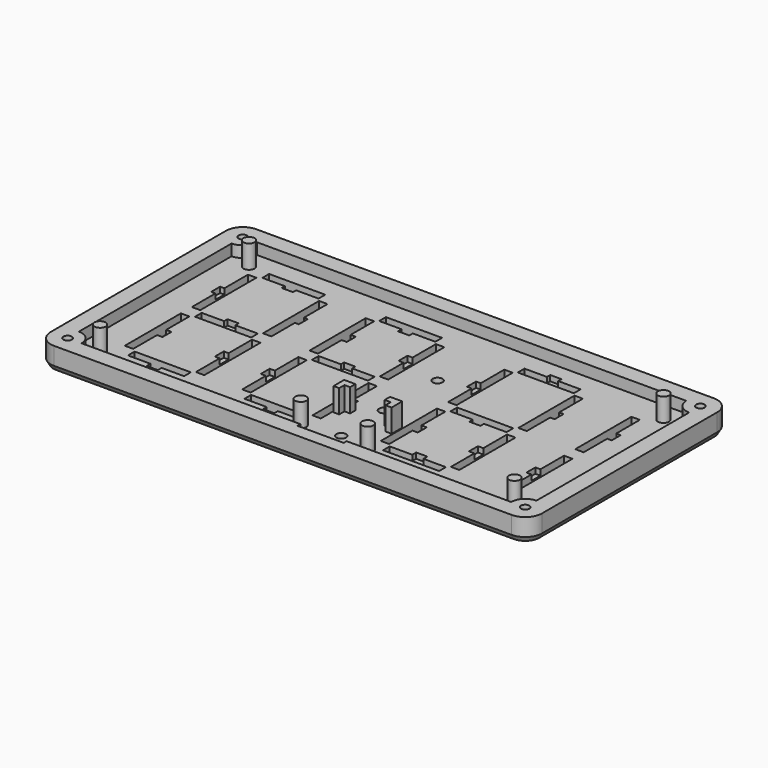
from build123d import *

# Parameters (mm, degrees)
F0_W     = 175
F0_H     = 90
F0_R     = 1.5
F0_R_2   = 2
F0_R_3   = 1.75
F0_W_2   = 16.51
F0_H_2   = 1.3014607364
F0_W_3   = 1.9210205078
F0_H_3   = 4
F0_W_4   = 1.9112368478
F0_W_5   = 1.867620334
F0_W_6   = 1.8335093537
F0_W_7   = 1.8196914813
F0_W_8   = 1.798794187
F0_H_4   = 3.9840501759
F0_W_9   = 1.7908662094
F0_W_10  = 4
F0_H_5   = 1.748018801
F0_W_11  = 1.7107389867
F0_H_6   = 1.7050467432
F0_W_12  = 1.6551189721
F0_H_7   = 1.612730462
F0_W_13  = 1.6000587711
F0_H_8   = 4.0289216264
F0_W_14  = 1.5901946127
F0_H_9   = 1.5753317512
F0_H_10  = 1.5676104019
F0_W_15  = 1.5668362754
F0_W_16  = 1.5211995589
F0_H_11  = 1.4929155913
F0_H_12  = 1.4762649832
F0_H_13  = 1.4190260208
F0_H_14  = 1.4116684069
F0_W_17  = 1.3783299625
F1_DEPTH = 4
F2_DEPTH = 4
F3_DEPTH = 4
F4_DEPTH = 2
F5_R     = 6
F6_SIZE2 = 1.7320508076
F6_SIZE  = 1
F8_DEPTH = 8.25


# Not quite as in the source:
# - a feature names something its author has since deleted; it is built from what else it names


with BuildPart() as f1:
    # F0 (on Top) → F1 (new body)
    with BuildSketch(Plane.XY):
        Rectangle(F0_W, F0_H)
        with Locations((-81.5, -39)):
            Circle(F0_R, mode=Mode.SUBTRACT)
        with Locations((81.5, -39)):
            Circle(F0_R, mode=Mode.SUBTRACT)
        with BuildLine():
            Line((-81.5, -34), (-81.5, 34))
            ThreePointArc((-81.5, 34), (-77.9644660941, 35.4644660941), (-76.5, 39))
            Line((-76.5, 39), (76.5, 39))
            ThreePointArc((76.5, 39), (77.9644660941, 35.4644660941), (81.5, 34))
            Line((81.5, 34), (81.5, -34))
            ThreePointArc((81.5, -34), (77.9644660941, -35.4644660941), (76.5, -39))
            Line((76.5, -39), (17.9069533545, -39))
            Line((17.9069533545, -39), (17.9069533545, -40.3014607364))
            Line((17.9069533545, -40.3014607364), (1.3969533545, -40.3014607364))
            Line((1.3969533545, -40.3014607364), (1.3969533545, -39))
            Line((1.3969533545, -39), (-76.5, -39))
            ThreePointArc((-76.5, -39), (-77.9644660941, -35.4644660941), (-81.5, -34))
        make_face(mode=Mode.SUBTRACT)
        with Locations((-81.5, 39)):
            Circle(F0_R, mode=Mode.SUBTRACT)
        with Locations((81.5, 39)):
            Circle(F0_R, mode=Mode.SUBTRACT)
        with BuildLine():
            ThreePointArc((-76.5, 39), (-77.9644660941, 35.4644660941), (-81.5, 34))
            Line((-81.5, 34), (-81.5, -34))
            ThreePointArc((-81.5, -34), (-77.9644660941, -35.4644660941), (-76.5, -39))
            Line((-76.5, -39), (1.3969533545, -39))
            Line((1.3969533545, -39), (17.9069533545, -39))
            Line((17.9069533545, -39), (76.5, -39))
            ThreePointArc((76.5, -39), (77.9644660941, -35.4644660941), (81.5, -34))
            Line((81.5, -34), (81.5, 34))
            ThreePointArc((81.5, 34), (77.9644660941, 35.4644660941), (76.5, 39))
            Line((76.5, 39), (-76.5, 39))
        make_face()
        with Locations((-74.491012668, -33.333260566)):
            Circle(F0_R_2, mode=Mode.SUBTRACT)
        Polygon((-66.6752069294, -27.6686349213), (-46.6752069294, -27.6686349213), (-46.6752069294, -30.6686349213), (-54.6752069294, -30.6686349213), (-54.6752069294, -32.3736816645), (-58.6752069294, -32.3736816645), (-58.6752069294, -30.6686349213), (-66.6752069294, -30.6686349213), align=None, mode=Mode.SUBTRACT)
        Polygon((-25.0613520422, -27.8102330678), (-5.0613520422, -27.8102330678), (-5.0613520422, -30.8102330678), (-13.1632021666, -30.8102330678), (-13.1632021666, -32.4229635298), (-17.1632021666, -32.4229635298), (-17.1632021666, -30.8102330678), (-25.0613520422, -30.8102330678), align=None, mode=Mode.SUBTRACT)
        with Locations((-2.9774932191, -33.333260566)):
            Circle(F0_R_2, mode=Mode.SUBTRACT)
        Polygon((-68.0133168949, -16.0233359784), (-68.0133168949, -26.6686349213), (-71.0133168949, -26.6686349213), (-71.0133168949, -1.6686349213), (-68.0133168949, -1.6686349213), (-68.0133168949, -12.0233359784), (-66.1020800471, -12.0233359784), (-66.1020800471, -16.0233359784), align=None, mode=Mode.SUBTRACT)
        Polygon((-45.6752069294, -12.0996839404), (-45.6752069294, -1.6686349213), (-42.6752069294, -1.6686349213), (-42.6752069294, -26.6686349213), (-45.6752069294, -26.6686349213), (-45.6752069294, -16.0996839404), (-47.3859459162, -16.0996839404), (-47.3859459162, -12.0996839404), align=None, mode=Mode.SUBTRACT)
        Polygon((-29.0613520422, -1.8102330678), (-26.0613520422, -1.8102330678), (-26.0613520422, -26.8102330678), (-29.0613520422, -26.8102330678), (-29.0613520422, -16.2864062117), (-30.8810435236, -16.2864062117), (-30.8810435236, -12.2864062117), (-29.0613520422, -12.2864062117), align=None, mode=Mode.SUBTRACT)
        Polygon((-4.0613520422, -26.8102330678), (-4.0613520422, -1.8102330678), (-1.0613520422, -1.8102330678), (-1.0613520422, -12.2331848519), (0.5054842331, -12.2331848519), (0.5054842331, -16.2331848519), (-1.0613520422, -16.2331848519), (-1.0613520422, -26.8102330678), align=None, mode=Mode.SUBTRACT)
        with Locations((9.8969533545, -31.4114607364)):
            Circle(F0_R_3, mode=Mode.SUBTRACT)
        with Locations((20.8698699123, -33.333260566)):
            Circle(F0_R_2, mode=Mode.SUBTRACT)
        Polygon((36.4340835214, -27.958609998), (44.4077534974, -27.958609998), (44.4077534974, -30.958609998), (24.4077534974, -30.958609998), (24.4077534974, -27.958609998), (32.4340835214, -27.958609998), (32.4340835214, -26.210591197), (36.4340835214, -26.210591197), align=None, mode=Mode.SUBTRACT)
        with Locations((73.1534102804, -33.333260566)):
            Circle(F0_R_2, mode=Mode.SUBTRACT)
        Polygon((1.3969533545, -19.3464607364), (1.3969533545, -21.7163469642), (-0.608429326, -21.7163469642), (-0.608429326, -16.9765745085), (3.4023360349, -16.9765745085), (3.4023360349, -19.3464607364), align=None, mode=Mode.SUBTRACT)
        Polygon((17.9069533545, -21.7163469642), (17.9069533545, -19.3464607364), (15.7326646149, -19.3464607364), (15.7326646149, -16.9765745085), (20.081242094, -16.9765745085), (20.081242094, -21.7163469642), align=None, mode=Mode.SUBTRACT)
        with Locations((9.6294777468, -12.0452046394)):
            Circle(F0_R_3, mode=Mode.SUBTRACT)
        Polygon((20.4077534974, -26.958609998), (20.4077534974, -1.958609998), (23.4077534974, -1.958609998), (23.4077534974, -12.5651864777), (25.2753738314, -12.5651864777), (25.2753738314, -16.5651864777), (23.4077534974, -16.5651864777), (23.4077534974, -26.958609998), align=None, mode=Mode.SUBTRACT)
        Polygon((24.4077534974, 2.041390002), (44.4077534974, 2.041390002), (44.4077534974, -0.958609998), (36.3806852102, -0.958609998), (36.3806852102, -2.5262203999), (32.3806852102, -2.5262203999), (32.3806852102, -0.958609998), (24.4077534974, -0.958609998), align=None, mode=Mode.SUBTRACT)
        Polygon((45.4077534974, -12.5448077023), (45.4077534974, -1.958609998), (48.4077534974, -1.958609998), (48.4077534974, -26.958609998), (45.4077534974, -26.958609998), (45.4077534974, -16.5448077023), (43.4867329895, -16.5448077023), (43.4867329895, -12.5448077023), align=None, mode=Mode.SUBTRACT)
        Polygon((65.7603075275, -12.5448077023), (65.7603075275, -2.0368327902), (68.7603075275, -2.0368327902), (68.7603075275, -27.0368327902), (65.7603075275, -27.0368327902), (65.7603075275, -16.5288578782), (63.9615133405, -16.5288578782), (63.9615133405, -12.5448077023), align=None, mode=Mode.SUBTRACT)
        Polygon((-54.6752069294, 2.1897669322), (-46.6752069294, 2.1897669322), (-46.6752069294, -0.8102330678), (-66.6752069294, -0.8102330678), (-66.6752069294, 2.1897669322), (-58.6752069294, 2.1897669322), (-58.6752069294, 3.6826825235), (-54.6752069294, 3.6826825235), align=None, mode=Mode.SUBTRACT)
        Polygon((-68.0133168949, 28.1897669322), (-68.0133168949, 3.1897669322), (-71.0133168949, 3.1897669322), (-71.0133168949, 13.6897669322), (-72.5345164537, 13.6897669322), (-72.5345164537, 17.6897669322), (-71.0133168949, 17.6897669322), (-71.0133168949, 28.1897669322), align=None, mode=Mode.SUBTRACT)
        Polygon((-13.103722319, 2.1897669322), (-5.0613520422, 2.1897669322), (-5.0613520422, -0.8102330678), (-25.0613520422, -0.8102330678), (-25.0613520422, 2.1897669322), (-17.103722319, 2.1897669322), (-17.103722319, 3.6014353391), (-13.103722319, 3.6014353391), align=None, mode=Mode.SUBTRACT)
        Polygon((-42.6752069294, 13.6755983604), (-42.6752069294, 3.1897669322), (-45.6752069294, 3.1897669322), (-45.6752069294, 28.1897669322), (-42.6752069294, 28.1897669322), (-42.6752069294, 17.6755983604), (-41.296876967, 17.6755983604), (-41.296876967, 13.6755983604), align=None, mode=Mode.SUBTRACT)
        Polygon((-29.0613520422, 28.1897669322), (-26.0613520422, 28.1897669322), (-26.0613520422, 17.6864017023), (-24.2278426886, 17.6864017023), (-24.2278426886, 13.6864017023), (-26.0613520422, 13.6864017023), (-26.0613520422, 3.1897669322), (-29.0613520422, 3.1897669322), align=None, mode=Mode.SUBTRACT)
        Polygon((-4.0613520422, 17.7803005055), (-4.0613520422, 28.1897669322), (-1.0613520422, 28.1897669322), (-1.0613520422, 3.1897669322), (-4.0613520422, 3.1897669322), (-4.0613520422, 13.7803005055), (-5.8522182517, 13.7803005055), (-5.8522182517, 17.7803005055), align=None, mode=Mode.SUBTRACT)
        with Locations((-73.842048645, 32.1897669322)):
            Circle(F0_R_2, mode=Mode.SUBTRACT)
        Polygon((-46.6752069294, 32.1897669322), (-46.6752069294, 29.1897669322), (-54.6752069294, 29.1897669322), (-54.6752069294, 27.7707409114), (-58.6752069294, 27.7707409114), (-58.6752069294, 29.1897669322), (-66.6752069294, 29.1897669322), (-66.6752069294, 32.1897669322), align=None, mode=Mode.SUBTRACT)
        Polygon((-5.0613520422, 32.1897669322), (-5.0613520422, 29.1897669322), (-13.1001572162, 29.1897669322), (-13.1001572162, 27.614435181), (-17.1001572162, 27.614435181), (-17.1001572162, 29.1897669322), (-25.0613520422, 29.1897669322), (-25.0613520422, 32.1897669322), align=None, mode=Mode.SUBTRACT)
        with Locations((10.0254695863, 11.318275705)):
            Circle(F0_R_3, mode=Mode.SUBTRACT)
        Polygon((23.4077534974, 28.041390002), (23.4077534974, 3.041390002), (20.4077534974, 3.041390002), (20.4077534974, 13.5473189875), (18.7526345253, 13.5473189875), (18.7526345253, 17.5473189875), (20.4077534974, 17.5473189875), (20.4077534974, 28.041390002), align=None, mode=Mode.SUBTRACT)
        Polygon((48.4077534974, 3.041390002), (45.4077534974, 3.041390002), (45.4077534974, 28.041390002), (48.4077534974, 28.041390002), (48.4077534974, 17.4776280229), (49.9979481101, 17.4776280229), (49.9979481101, 13.4776280229), (48.4077534974, 13.4776280229), align=None, mode=Mode.SUBTRACT)
        Polygon((68.7603075275, 2.9631672098), (65.7603075275, 2.9631672098), (65.7603075275, 27.9631672098), (68.7603075275, 27.9631672098), (68.7603075275, 17.4776280229), (70.3603662986, 17.4776280229), (70.3603662986, 13.4487063966), (68.7603075275, 13.4487063966), align=None, mode=Mode.SUBTRACT)
        Polygon((36.4043445289, 32.041390002), (44.4077534974, 32.041390002), (44.4077534974, 29.041390002), (24.4077534974, 29.041390002), (24.4077534974, 32.041390002), (32.4043445289, 32.041390002), (32.4043445289, 33.5176549852), (36.4043445289, 33.5176549852), align=None, mode=Mode.SUBTRACT)
        with Locations((73.8023817539, 32.1897669322)):
            Circle(F0_R_2, mode=Mode.SUBTRACT)
        Polygon((-1.0613520422, 28.1897669322), (-4.0613520422, 28.1897669322), (-4.0613520422, 17.7803005055), (-4.0613520422, 13.7803005055), (-4.0613520422, 3.1897669322), (-1.0613520422, 3.1897669322), align=None)
        Polygon((-1.0613520422, -1.8102330678), (-4.0613520422, -1.8102330678), (-4.0613520422, -26.8102330678), (-1.0613520422, -26.8102330678), (-1.0613520422, -16.2331848519), (-1.0613520422, -12.2331848519), align=None)
        Polygon((48.4077534974, -1.958609998), (45.4077534974, -1.958609998), (45.4077534974, -12.5448077023), (45.4077534974, -16.5448077023), (45.4077534974, -26.958609998), (48.4077534974, -26.958609998), align=None)
        Polygon((-71.0133168949, -26.6686349213), (-68.0133168949, -26.6686349213), (-68.0133168949, -16.0233359784), (-68.0133168949, -12.0233359784), (-68.0133168949, -1.6686349213), (-71.0133168949, -1.6686349213), align=None)
        Polygon((-71.0133168949, 3.1897669322), (-68.0133168949, 3.1897669322), (-68.0133168949, 28.1897669322), (-71.0133168949, 28.1897669322), (-71.0133168949, 17.6897669322), (-71.0133168949, 13.6897669322), align=None)
        Polygon((-42.6752069294, -1.6686349213), (-45.6752069294, -1.6686349213), (-45.6752069294, -12.0996839404), (-45.6752069294, -16.0996839404), (-45.6752069294, -26.6686349213), (-42.6752069294, -26.6686349213), align=None)
        Polygon((-45.6752069294, 3.1897669322), (-42.6752069294, 3.1897669322), (-42.6752069294, 13.6755983604), (-42.6752069294, 17.6755983604), (-42.6752069294, 28.1897669322), (-45.6752069294, 28.1897669322), align=None)
        Polygon((65.7603075275, 27.9631672098), (65.7603075275, 2.9631672098), (68.7603075275, 2.9631672098), (68.7603075275, 13.4487063966), (68.7603075275, 17.4776280229), (68.7603075275, 27.9631672098), align=None)
        Polygon((20.4077534974, 3.041390002), (23.4077534974, 3.041390002), (23.4077534974, 28.041390002), (20.4077534974, 28.041390002), (20.4077534974, 17.5473189875), (20.4077534974, 13.5473189875), align=None)
        Polygon((23.4077534974, -1.958609998), (20.4077534974, -1.958609998), (20.4077534974, -26.958609998), (23.4077534974, -26.958609998), (23.4077534974, -16.5651864777), (23.4077534974, -12.5651864777), align=None)
        Polygon((68.7603075275, -2.0368327902), (65.7603075275, -2.0368327902), (65.7603075275, -12.5448077023), (65.7603075275, -16.5288578782), (65.7603075275, -27.0368327902), (68.7603075275, -27.0368327902), align=None)
        Polygon((-26.0613520422, -26.8102330678), (-26.0613520422, -1.8102330678), (-29.0613520422, -1.8102330678), (-29.0613520422, -12.2864062117), (-29.0613520422, -16.2864062117), (-29.0613520422, -26.8102330678), align=None)
        Polygon((-26.0613520422, 17.6864017023), (-26.0613520422, 28.1897669322), (-29.0613520422, 28.1897669322), (-29.0613520422, 3.1897669322), (-26.0613520422, 3.1897669322), (-26.0613520422, 13.6864017023), align=None)
        Polygon((45.4077534974, 28.041390002), (45.4077534974, 3.041390002), (48.4077534974, 3.041390002), (48.4077534974, 13.4776280229), (48.4077534974, 17.4776280229), (48.4077534974, 28.041390002), align=None)
        Polygon((-5.0613520422, -30.8102330678), (-5.0613520422, -27.8102330678), (-25.0613520422, -27.8102330678), (-25.0613520422, -30.8102330678), (-17.1632021666, -30.8102330678), (-13.1632021666, -30.8102330678), align=None)
        Polygon((-46.6752069294, -30.6686349213), (-46.6752069294, -27.6686349213), (-66.6752069294, -27.6686349213), (-66.6752069294, -30.6686349213), (-58.6752069294, -30.6686349213), (-54.6752069294, -30.6686349213), align=None)
        Polygon((44.4077534974, -0.958609998), (44.4077534974, 2.041390002), (24.4077534974, 2.041390002), (24.4077534974, -0.958609998), (32.3806852102, -0.958609998), (36.3806852102, -0.958609998), align=None)
        Polygon((44.4077534974, -30.958609998), (44.4077534974, -27.958609998), (36.4340835214, -27.958609998), (32.4340835214, -27.958609998), (24.4077534974, -27.958609998), (24.4077534974, -30.958609998), align=None)
        Polygon((-54.6752069294, 29.1897669322), (-46.6752069294, 29.1897669322), (-46.6752069294, 32.1897669322), (-66.6752069294, 32.1897669322), (-66.6752069294, 29.1897669322), (-58.6752069294, 29.1897669322), align=None)
        Polygon((-46.6752069294, -0.8102330678), (-46.6752069294, 2.1897669322), (-54.6752069294, 2.1897669322), (-58.6752069294, 2.1897669322), (-66.6752069294, 2.1897669322), (-66.6752069294, -0.8102330678), align=None)
        Polygon((-5.0613520422, -0.8102330678), (-5.0613520422, 2.1897669322), (-13.103722319, 2.1897669322), (-17.103722319, 2.1897669322), (-25.0613520422, 2.1897669322), (-25.0613520422, -0.8102330678), align=None)
        Polygon((-13.1001572162, 29.1897669322), (-5.0613520422, 29.1897669322), (-5.0613520422, 32.1897669322), (-25.0613520422, 32.1897669322), (-25.0613520422, 29.1897669322), (-17.1001572162, 29.1897669322), align=None)
        Polygon((44.4077534974, 29.041390002), (44.4077534974, 32.041390002), (36.4043445289, 32.041390002), (32.4043445289, 32.041390002), (24.4077534974, 32.041390002), (24.4077534974, 29.041390002), align=None)
        with Locations((9.6519533545, -39.6507303682)):
            Rectangle(F0_W_2, F0_H_2)
        Polygon((15.7326646149, -19.3464607364), (17.9069533545, -19.3464607364), (17.9069533545, -21.7163469642), (20.081242094, -21.7163469642), (20.081242094, -16.9765745085), (15.7326646149, -16.9765745085), align=None)
        Polygon((-0.608429326, -21.7163469642), (1.3969533545, -21.7163469642), (1.3969533545, -19.3464607364), (3.4023360349, -19.3464607364), (3.4023360349, -16.9765745085), (-0.608429326, -16.9765745085), align=None)
        with Locations((73.8023817539, 32.1897669322)):
            Circle(F0_R_2)
        with Locations((73.1534102804, -33.333260566)):
            Circle(F0_R_2)
        with Locations((-74.491012668, -33.333260566)):
            Circle(F0_R_2)
        with Locations((-73.842048645, 32.1897669322)):
            Circle(F0_R_2)
        with Locations((-2.9774932191, -33.333260566)):
            Circle(F0_R_2)
        with Locations((20.8698699123, -33.333260566)):
            Circle(F0_R_2)
        with Locations((9.6294777468, -12.0452046394)):
            Circle(F0_R_3)
        with Locations((10.0254695863, 11.318275705)):
            Circle(F0_R_3)
        with Locations((9.8969533545, -31.4114607364)):
            Circle(F0_R_3)
        with Locations((44.4472432435, -14.5448077023)):
            Rectangle(F0_W_3, F0_H_3)
        with Locations((-67.057698471, -14.0233359784)):
            Rectangle(F0_W_4, F0_H_3)
        with Locations((24.3415636644, -14.5651864777)):
            Rectangle(F0_W_5, F0_H_3)
        with Locations((-25.1445973654, 15.6864017023)):
            Rectangle(F0_W_6, F0_H_3)
        with Locations((-29.9711977829, -14.2864062117)):
            Rectangle(F0_W_7, F0_H_3)
        with Locations((64.860910434, -14.5368327902)):
            Rectangle(F0_W_8, F0_H_4)
        with Locations((-4.956785147, 15.7803005055)):
            Rectangle(F0_W_9, F0_H_3)
        with Locations((-81.5, 39)):
            Circle(F0_R)
        with Locations((-81.5, -39)):
            Circle(F0_R)
        with Locations((81.5, -39)):
            Circle(F0_R)
        with Locations((81.5, 39)):
            Circle(F0_R)
        with Locations((34.4340835214, -27.0846005975)):
            Rectangle(F0_W_10, F0_H_5)
        with Locations((-46.5305764228, -14.0996839404)):
            Rectangle(F0_W_11, F0_H_3)
        with Locations((-56.6752069294, -31.5211582929)):
            Rectangle(F0_W_10, F0_H_6)
        with Locations((19.5801940113, 15.5473189875)):
            Rectangle(F0_W_12, F0_H_3)
        with Locations((-15.1632021666, -31.6165982988)):
            Rectangle(F0_W_10, F0_H_7)
        with Locations((69.5603369131, 15.4631672098)):
            Rectangle(F0_W_13, F0_H_8)
        with Locations((49.2028508037, 15.4776280229)):
            Rectangle(F0_W_14, F0_H_3)
        with Locations((-15.1001572162, 28.4021010566)):
            Rectangle(F0_W_10, F0_H_9)
        with Locations((34.3806852102, -1.7424151989)):
            Rectangle(F0_W_10, F0_H_10)
        with Locations((-0.2779339045, -14.2331848519)):
            Rectangle(F0_W_15, F0_H_3)
        with Locations((-71.7739166743, 15.6897669322)):
            Rectangle(F0_W_16, F0_H_3)
        with Locations((-56.6752069294, 2.9362247278)):
            Rectangle(F0_W_10, F0_H_11)
        with Locations((34.4043445289, 32.7795224936)):
            Rectangle(F0_W_10, F0_H_12)
        with Locations((-56.6752069294, 28.4802539218)):
            Rectangle(F0_W_10, F0_H_13)
        with Locations((-15.103722319, 2.8956011356)):
            Rectangle(F0_W_10, F0_H_14)
        with Locations((-41.9860419482, 15.6755983604)):
            Rectangle(F0_W_17, F0_H_3)
    extrude(amount=-F1_DEPTH)

    # F0 (on Top) → F2 (join)
    with BuildSketch(Plane.XY):
        Rectangle(F0_W, F0_H)
        with Locations((-81.5, -39)):
            Circle(F0_R, mode=Mode.SUBTRACT)
        with Locations((81.5, -39)):
            Circle(F0_R, mode=Mode.SUBTRACT)
        with BuildLine():
            Line((-81.5, -34), (-81.5, 34))
            ThreePointArc((-81.5, 34), (-77.9644660941, 35.4644660941), (-76.5, 39))
            Line((-76.5, 39), (76.5, 39))
            ThreePointArc((76.5, 39), (77.9644660941, 35.4644660941), (81.5, 34))
            Line((81.5, 34), (81.5, -34))
            ThreePointArc((81.5, -34), (77.9644660941, -35.4644660941), (76.5, -39))
            Line((76.5, -39), (17.9069533545, -39))
            Line((17.9069533545, -39), (17.9069533545, -40.3014607364))
            Line((17.9069533545, -40.3014607364), (1.3969533545, -40.3014607364))
            Line((1.3969533545, -40.3014607364), (1.3969533545, -39))
            Line((1.3969533545, -39), (-76.5, -39))
            ThreePointArc((-76.5, -39), (-77.9644660941, -35.4644660941), (-81.5, -34))
        make_face(mode=Mode.SUBTRACT)
        with Locations((-81.5, 39)):
            Circle(F0_R, mode=Mode.SUBTRACT)
        with Locations((81.5, 39)):
            Circle(F0_R, mode=Mode.SUBTRACT)
    extrude(amount=F2_DEPTH)

    # F0 (on Top) → F3 (cut)
    with BuildSketch(Plane.XY):
        Polygon((-54.6752069294, 29.1897669322), (-46.6752069294, 29.1897669322), (-46.6752069294, 32.1897669322), (-66.6752069294, 32.1897669322), (-66.6752069294, 29.1897669322), (-58.6752069294, 29.1897669322), align=None)
        Polygon((-71.0133168949, 3.1897669322), (-68.0133168949, 3.1897669322), (-68.0133168949, 28.1897669322), (-71.0133168949, 28.1897669322), (-71.0133168949, 17.6897669322), (-71.0133168949, 13.6897669322), align=None)
        Polygon((-45.6752069294, 3.1897669322), (-42.6752069294, 3.1897669322), (-42.6752069294, 13.6755983604), (-42.6752069294, 17.6755983604), (-42.6752069294, 28.1897669322), (-45.6752069294, 28.1897669322), align=None)
        Polygon((-46.6752069294, -0.8102330678), (-46.6752069294, 2.1897669322), (-54.6752069294, 2.1897669322), (-58.6752069294, 2.1897669322), (-66.6752069294, 2.1897669322), (-66.6752069294, -0.8102330678), align=None)
        Polygon((-42.6752069294, -1.6686349213), (-45.6752069294, -1.6686349213), (-45.6752069294, -12.0996839404), (-45.6752069294, -16.0996839404), (-45.6752069294, -26.6686349213), (-42.6752069294, -26.6686349213), align=None)
        Polygon((-71.0133168949, -26.6686349213), (-68.0133168949, -26.6686349213), (-68.0133168949, -16.0233359784), (-68.0133168949, -12.0233359784), (-68.0133168949, -1.6686349213), (-71.0133168949, -1.6686349213), align=None)
        Polygon((-46.6752069294, -30.6686349213), (-46.6752069294, -27.6686349213), (-66.6752069294, -27.6686349213), (-66.6752069294, -30.6686349213), (-58.6752069294, -30.6686349213), (-54.6752069294, -30.6686349213), align=None)
        Polygon((-26.0613520422, 17.6864017023), (-26.0613520422, 28.1897669322), (-29.0613520422, 28.1897669322), (-29.0613520422, 3.1897669322), (-26.0613520422, 3.1897669322), (-26.0613520422, 13.6864017023), align=None)
        Polygon((-13.1001572162, 29.1897669322), (-5.0613520422, 29.1897669322), (-5.0613520422, 32.1897669322), (-25.0613520422, 32.1897669322), (-25.0613520422, 29.1897669322), (-17.1001572162, 29.1897669322), align=None)
        Polygon((-1.0613520422, 28.1897669322), (-4.0613520422, 28.1897669322), (-4.0613520422, 17.7803005055), (-4.0613520422, 13.7803005055), (-4.0613520422, 3.1897669322), (-1.0613520422, 3.1897669322), align=None)
        Polygon((-5.0613520422, -0.8102330678), (-5.0613520422, 2.1897669322), (-13.103722319, 2.1897669322), (-17.103722319, 2.1897669322), (-25.0613520422, 2.1897669322), (-25.0613520422, -0.8102330678), align=None)
        Polygon((-26.0613520422, -26.8102330678), (-26.0613520422, -1.8102330678), (-29.0613520422, -1.8102330678), (-29.0613520422, -12.2864062117), (-29.0613520422, -16.2864062117), (-29.0613520422, -26.8102330678), align=None)
        Polygon((-5.0613520422, -30.8102330678), (-5.0613520422, -27.8102330678), (-25.0613520422, -27.8102330678), (-25.0613520422, -30.8102330678), (-17.1632021666, -30.8102330678), (-13.1632021666, -30.8102330678), align=None)
        Polygon((-1.0613520422, -1.8102330678), (-4.0613520422, -1.8102330678), (-4.0613520422, -26.8102330678), (-1.0613520422, -26.8102330678), (-1.0613520422, -16.2331848519), (-1.0613520422, -12.2331848519), align=None)
        with Locations((10.0254695863, 11.318275705)):
            Circle(F0_R_3)
        with Locations((9.6294777468, -12.0452046394)):
            Circle(F0_R_3)
        Polygon((23.4077534974, -1.958609998), (20.4077534974, -1.958609998), (20.4077534974, -26.958609998), (23.4077534974, -26.958609998), (23.4077534974, -16.5651864777), (23.4077534974, -12.5651864777), align=None)
        Polygon((20.4077534974, 3.041390002), (23.4077534974, 3.041390002), (23.4077534974, 28.041390002), (20.4077534974, 28.041390002), (20.4077534974, 17.5473189875), (20.4077534974, 13.5473189875), align=None)
        Polygon((44.4077534974, -0.958609998), (44.4077534974, 2.041390002), (24.4077534974, 2.041390002), (24.4077534974, -0.958609998), (32.3806852102, -0.958609998), (36.3806852102, -0.958609998), align=None)
        Polygon((45.4077534974, 28.041390002), (45.4077534974, 3.041390002), (48.4077534974, 3.041390002), (48.4077534974, 13.4776280229), (48.4077534974, 17.4776280229), (48.4077534974, 28.041390002), align=None)
        Polygon((44.4077534974, 29.041390002), (44.4077534974, 32.041390002), (36.4043445289, 32.041390002), (32.4043445289, 32.041390002), (24.4077534974, 32.041390002), (24.4077534974, 29.041390002), align=None)
        Polygon((65.7603075275, 27.9631672098), (65.7603075275, 2.9631672098), (68.7603075275, 2.9631672098), (68.7603075275, 13.4487063966), (68.7603075275, 17.4776280229), (68.7603075275, 27.9631672098), align=None)
        Polygon((68.7603075275, -2.0368327902), (65.7603075275, -2.0368327902), (65.7603075275, -12.5448077023), (65.7603075275, -16.5288578782), (65.7603075275, -27.0368327902), (68.7603075275, -27.0368327902), align=None)
        Polygon((48.4077534974, -1.958609998), (45.4077534974, -1.958609998), (45.4077534974, -12.5448077023), (45.4077534974, -16.5448077023), (45.4077534974, -26.958609998), (48.4077534974, -26.958609998), align=None)
        Polygon((44.4077534974, -30.958609998), (44.4077534974, -27.958609998), (36.4340835214, -27.958609998), (32.4340835214, -27.958609998), (24.4077534974, -27.958609998), (24.4077534974, -30.958609998), align=None)
        with Locations((9.8969533545, -31.4114607364)):
            Circle(F0_R_3)
    extrude(amount=-F3_DEPTH, mode=Mode.SUBTRACT)

    # F0 (on Top) → F4 (cut)
    with BuildSketch(Plane.XY):
        with Locations((-15.1001572162, 28.4021010566)):
            Rectangle(F0_W_10, F0_H_9)
        with Locations((-4.956785147, 15.7803005055)):
            Rectangle(F0_W_9, F0_H_3)
        with Locations((-25.1445973654, 15.6864017023)):
            Rectangle(F0_W_6, F0_H_3)
        with Locations((19.5801940113, 15.5473189875)):
            Rectangle(F0_W_12, F0_H_3)
        with Locations((34.4043445289, 32.7795224936)):
            Rectangle(F0_W_10, F0_H_12)
        with Locations((49.2028508037, 15.4776280229)):
            Rectangle(F0_W_14, F0_H_3)
        with Locations((69.5603369131, 15.4631672098)):
            Rectangle(F0_W_13, F0_H_8)
        with Locations((64.860910434, -14.5368327902)):
            Rectangle(F0_W_8, F0_H_4)
        with Locations((44.4472432435, -14.5448077023)):
            Rectangle(F0_W_3, F0_H_3)
        with Locations((34.3806852102, -1.7424151989)):
            Rectangle(F0_W_10, F0_H_10)
        with Locations((24.3415636644, -14.5651864777)):
            Rectangle(F0_W_5, F0_H_3)
        with Locations((34.4340835214, -27.0846005975)):
            Rectangle(F0_W_10, F0_H_5)
        with Locations((-0.2779339045, -14.2331848519)):
            Rectangle(F0_W_15, F0_H_3)
        with Locations((-15.1632021666, -31.6165982988)):
            Rectangle(F0_W_10, F0_H_7)
        with Locations((-29.9711977829, -14.2864062117)):
            Rectangle(F0_W_7, F0_H_3)
        with Locations((-15.103722319, 2.8956011356)):
            Rectangle(F0_W_10, F0_H_14)
        with Locations((-71.7739166743, 15.6897669322)):
            Rectangle(F0_W_16, F0_H_3)
        with Locations((-56.6752069294, 28.4802539218)):
            Rectangle(F0_W_10, F0_H_13)
        with Locations((-41.9860419482, 15.6755983604)):
            Rectangle(F0_W_17, F0_H_3)
        with Locations((-46.5305764228, -14.0996839404)):
            Rectangle(F0_W_11, F0_H_3)
        with Locations((-56.6752069294, 2.9362247278)):
            Rectangle(F0_W_10, F0_H_11)
        with Locations((-67.057698471, -14.0233359784)):
            Rectangle(F0_W_4, F0_H_3)
        with Locations((-56.6752069294, -31.5211582929)):
            Rectangle(F0_W_10, F0_H_6)
    extrude(amount=-F4_DEPTH, mode=Mode.SUBTRACT)

    # F5
    f5_edges = [f1.edges().sort_by_distance(p)[0] for p in [
        (87.5, -45, 0),
        (87.5, 45, 0),
        (-87.5, -45, 0),
        (-87.5, 45, 0),
    ]]
    fillet(f5_edges, radius=F5_R)

    # F6
    f6_edges = [f1.edges().sort_by_distance(p)[0] for p in [
        (87.5, 0, -4),
    ]]
    f6_side = f1.faces().sort_by_distance((0.538656, -0.050499, -4))[0]
    chamfer(f6_edges, length=F6_SIZE, length2=F6_SIZE2, reference=f6_side)

    # F0 (on Top) → F8 (join)
    with BuildSketch(Plane.XY):
        with Locations((-74.491012668, -33.333260566)):
            Circle(F0_R_2)
        with Locations((-2.9774932191, -33.333260566)):
            Circle(F0_R_2)
        Polygon((-0.608429326, -21.7163469642), (1.3969533545, -21.7163469642), (1.3969533545, -19.3464607364), (3.4023360349, -19.3464607364), (3.4023360349, -16.9765745085), (-0.608429326, -16.9765745085), align=None)
        Polygon((15.7326646149, -19.3464607364), (17.9069533545, -19.3464607364), (17.9069533545, -21.7163469642), (20.081242094, -21.7163469642), (20.081242094, -16.9765745085), (15.7326646149, -16.9765745085), align=None)
        with Locations((20.8698699123, -33.333260566)):
            Circle(F0_R_2)
        with Locations((73.1534102804, -33.333260566)):
            Circle(F0_R_2)
        with Locations((73.8023817539, 32.1897669322)):
            Circle(F0_R_2)
        with Locations((-73.842048645, 32.1897669322)):
            Circle(F0_R_2)
    extrude(amount=F8_DEPTH)


solid = f1.part
